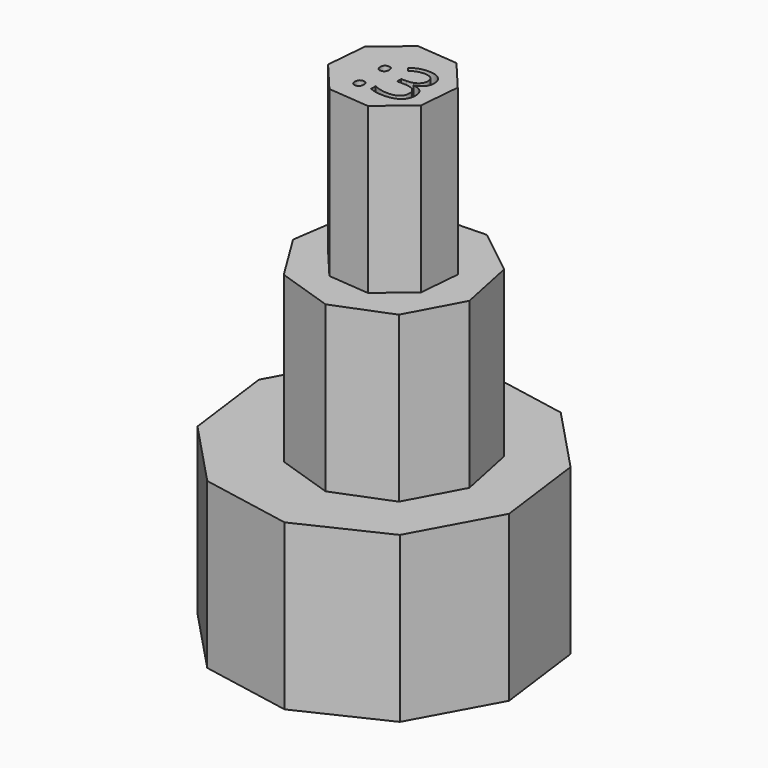
from build123d import *

# Parameters (mm, degrees)
F1_DEPTH      = 13.97
F3_DEPTH      = 27.94
F5_DEPTH      = 41.91
F6_TEXT_SIZE  = 6.2397871968
F7_DEPTH      = 7.62
F7_DEPTH_BACK = 25.4


# Not quite as in the source:
# - Text() gives the source's letters only with a copy of the font that has no kerning and outlines rounded to 1/6400 em; it was checked with that copy


with BuildPart() as f1:
    # F0 (on Top) → F1 (new body)
    with BuildSketch(Plane.XY):
        Polygon((7.9692486091, -9.2267929405), (11.7259590973, -2.3351730829), (10.7144092084, 5.4484035228), (5.3209766188, 11.1508751672), (-2.3942307385, 12.5940915021), (-9.4842658831, 9.2267929405), (-13.2409763713, 2.3351730829), (-12.2294264825, -5.4484035228), (-6.8359938928, -11.1508751672), (0.8792134645, -12.5940915021), align=None)
    extrude(amount=F1_DEPTH)

    # F2 (on Top) → F3 (join)
    with BuildSketch(Plane.XY):
        Polygon((4.9386678692, -5.5431868651), (7.3463309127, -1.0718129805), (6.3165640768, 3.9010741096), (2.3312067085, 7.0486052682), (-2.7449481872, 6.8980156853), (-6.5367113193, 3.5197679003), (-7.2698745778, -1.5054184031), (-4.6013827256, -5.8262027048), (0.2201472426, -7.4208420099), align=None)
    extrude(amount=F3_DEPTH)

    # F4 (on Top) → F5 (join)
    with BuildSketch(Plane.XY):
        Polygon((4.3912308358, 1.3870998945), (2.1242413602, 4.0858968433), (-1.3870998945, 4.3912308358), (-4.0858968433, 2.1242413602), (-4.3912308358, -1.3870998945), (-2.1242413602, -4.0858968433), (1.3870998945, -4.3912308358), (4.0858968433, -2.1242413602), align=None)
    extrude(amount=F5_DEPTH)

    # F6 (on face) → F7 (cut, two sides)
    with BuildSketch(Plane.XY.offset(41.91)) as f7_sk:
        with Locations((-1.9280061824, -2.5129320566)):
            Text(':3', F6_TEXT_SIZE, font='Open Sans', text_align=(TextAlign.LEFT, TextAlign.BOTTOM))
    extrude(amount=-F7_DEPTH, mode=Mode.SUBTRACT)
    extrude(f7_sk.sketch, amount=F7_DEPTH_BACK, mode=Mode.SUBTRACT)


solid = f1.part
